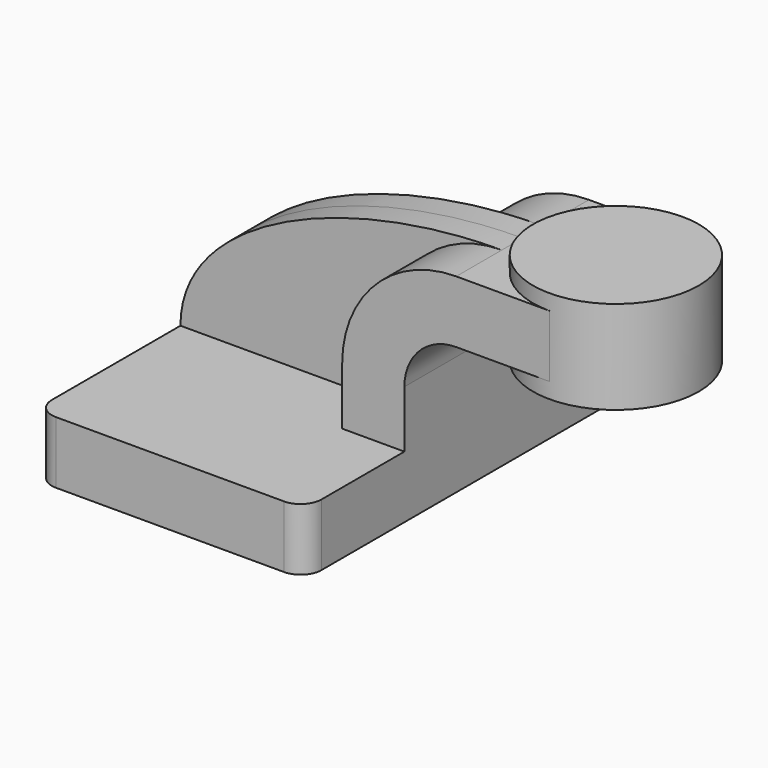
from build123d import *

# Parameters (mm, degrees)
F1_DEPTH = 63.5
F0_W     = 25.4
F0_H     = 19.05
F2_DEPTH = 25.4
F3_DEPTH = 7.9375
F5_R     = 6.35


# Not quite as in the source:
# - a feature names something its author has since deleted; it is built from what else it names


with BuildPart() as f1:
    # F0 (on Front) → F1 (new body, symmetric)
    with BuildSketch(Plane.XZ):
        Polygon((-41.275, 9.525), (-41.275, -9.525), (41.275, -9.525), (41.275, 9.525), (22.225, 9.525), align=None)
    extrude(amount=F1_DEPTH, both=True)

    # F0 (on Front) → F2 (join, symmetric)
    with BuildSketch(Plane.XZ):
        with BuildLine():
            Line((22.225, 9.525), (41.275, 9.525))
            Line((41.275, 9.525), (41.275, 27.0002))
            ThreePointArc((41.275, 27.0002), (45.9246798487, 38.2255201513), (57.15, 42.8752))
            Line((57.15, 42.8752), (60.325, 42.8752))
            Line((60.325, 42.8752), (60.325, 61.9252))
            Line((60.325, 61.9252), (57.15, 61.9252))
            ThreePointArc((57.15, 61.9252), (32.4542956671, 51.6959043329), (22.225, 27.0002))
            Line((22.225, 27.0002), (22.225, 9.525))
        make_face()
        with Locations((73.025, 52.4002)):
            Rectangle(F0_W, F0_H)
    extrude(amount=F2_DEPTH, both=True)

    # F0 (on Front) → F3 (join, symmetric)
    with BuildSketch(Plane.XZ):
        with BuildLine():
            add(Edge.make_bspline(
                [(-41.275, 9.525), (-41.275, 40.5423477454), (8.4285710651, 61.9252), (57.15, 61.9252)],
                knots=[0, 0, 0, 0, 111.5045361635, 111.5045361635, 111.5045361635, 111.5045361635], degree=3))
            Line((-41.275, 9.525), (22.225, 9.525))
            Line((22.225, 9.525), (22.225, 27.0002))
            ThreePointArc((22.225, 27.0002), (32.4542956671, 51.6959043329), (57.15, 61.9252))
        make_face()
    extrude(amount=F3_DEPTH, both=True)

    # F0 (on Front) → F4 (revolve)
    with BuildSketch(Plane.XZ):
        Polygon((85.725, 66.675), (85.725, 61.9252), (85.725, 42.8752), (85.725, 38.1), (111.125, 38.1), (111.125, 66.675), align=None)
    revolve(axis=Axis((85.725, 0, 52.3875), (0, 0, 1)))

    # F5
    f5_edges = [f1.edges().sort_by_distance(p)[0] for p in [
        (41.275, -63.5, 0),
        (-41.275, -63.5, 0),
        (41.275, 63.5, 0),
        (-41.275, 63.5, 0),
    ]]
    fillet(f5_edges, radius=F5_R)


solid = f1.part
